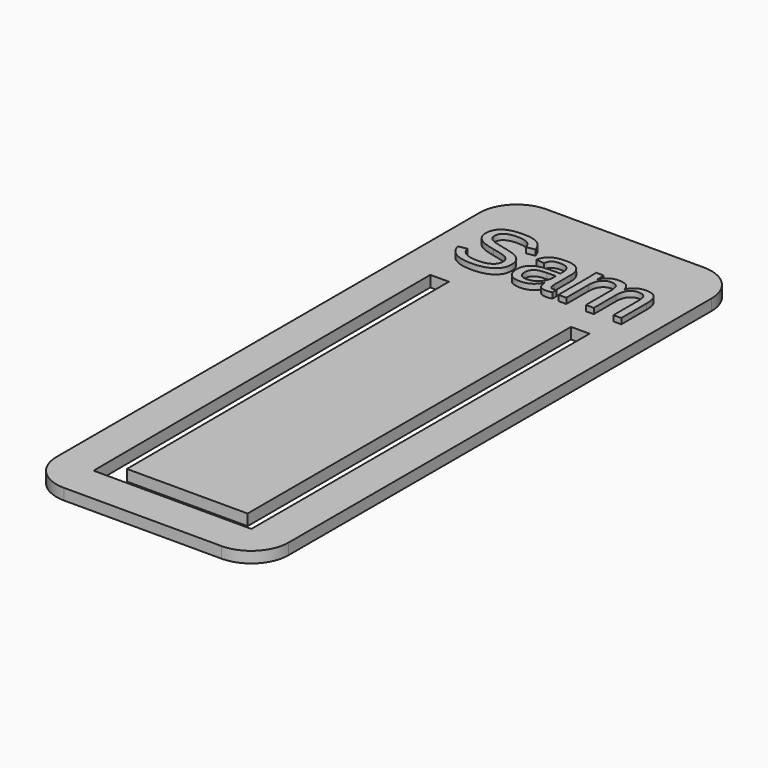
from build123d import *

# Parameters (mm, degrees)
F1_DEPTH     = 1.2
F2_TEXT_SIZE = 9.7109475761
F3_DEPTH     = 1.8


# Not quite as in the source:
# - Text() gives the source's letters only with a copy of the font that has no kerning and outlines rounded to 1/6400 em; it was checked with that copy


with BuildPart() as f1:
    # F0 (on Top) → F1 (new body)
    with BuildSketch(Plane.XY):
        with BuildLine():
            Line((9.9163665473, 28.1831063433), (-7.0836334527, 28.1831063433))
            ThreePointArc((-7.0836334527, 28.1831063433), (-9.9120605774, 27.011533468), (-11.0836334527, 24.1831063433))
            Line((-11.0836334527, 24.1831063433), (-11.0836334527, -32.8168936567))
            ThreePointArc((-11.0836334527, -32.8168936567), (-9.9120605774, -35.6453207815), (-7.0836334527, -36.8168936567))
            Line((-7.0836334527, -36.8168936567), (9.9163665473, -36.8168936567))
            ThreePointArc((9.9163665473, -36.8168936567), (12.7447936721, -35.6453207815), (13.9163665473, -32.8168936567))
            Line((13.9163665473, -32.8168936567), (13.9163665473, 24.1831063433))
            ThreePointArc((13.9163665473, 24.1831063433), (12.7447936721, 27.011533468), (9.9163665473, 28.1831063433))
        make_face()
        Polygon((-7.0836334527, -32.8168936567), (-7.2489720769, 12.7457063645), (-5.2489852452, 12.7529639633), (-5.0908779309, -30.8168936567), (7.9163665473, -30.8168936567), (7.9163665473, 12.7457063645), (9.9163665473, 12.7457063645), (9.9163665473, -32.8168936567), align=None, mode=Mode.SUBTRACT)
    extrude(amount=F1_DEPTH)

    # F2 (on Top) → F3 (join)
    with BuildSketch(Plane.XY):
        with Locations((-8.3910409949, 15.7468553869)):
            Text('Sam', F2_TEXT_SIZE, font='Arimo', text_align=(TextAlign.LEFT, TextAlign.BOTTOM))
    extrude(amount=F3_DEPTH)


solid = f1.part
